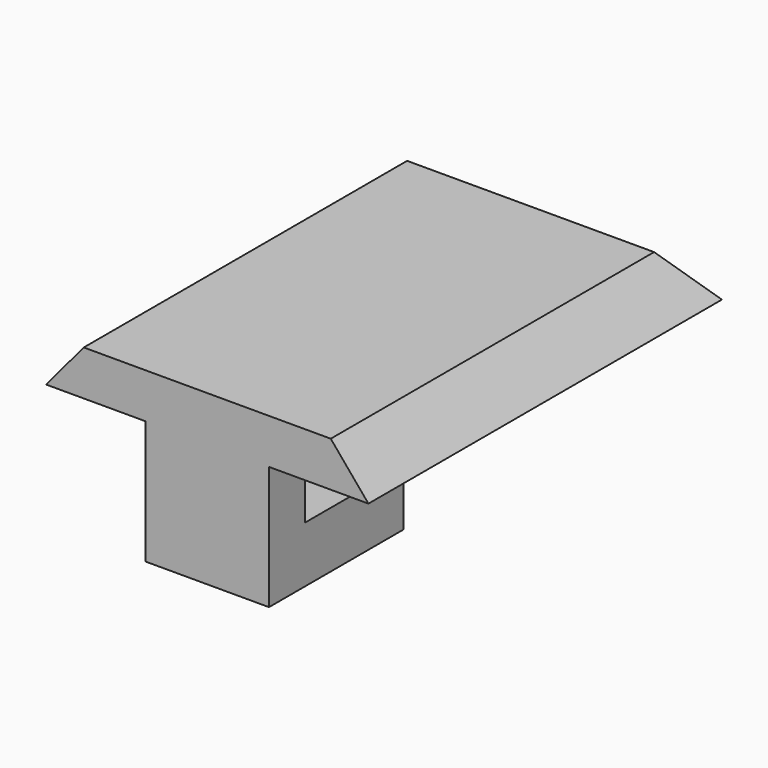
from build123d import *

# Parameters (mm, degrees)
F1_DEPTH    = 5.5
F2_DEPTH    = 15
F3_T1_DEPTH = 64.5730638659
F3_T3_DEPTH = 54.5730638659


# Not quite as in the source:
# - a fillet or chamfer that OpenCascade refuses, or shapes differently, is made with other operations: its cross-section is extruded or revolved along the edge and cut away or added


with BuildPart() as f1:
    # F0 (on Right) → F1 (new body, symmetric)
    with BuildSketch(Plane.YZ):
        Polygon((-11, 0), (0, 0), (0, 5), (-11, 5), (-11, 11), (-15, 11), (-15, 0), align=None)
    extrude(amount=F1_DEPTH, both=True)

    # F0 (on Right) → F2 (join, symmetric)
    with BuildSketch(Plane.YZ):
        Polygon((-15, 15), (-15, 11), (-11, 11), (25, 11), (25, 15), align=None)
    extrude(amount=F2_DEPTH, both=True)

    # F3: chamfer of 4 x 4.7670143704 on 3 edges, made by hand

    # F3_s2 → F3_t1 (cut)
    with BuildSketch(Plane.XZ.offset(-37.2865319329)):
        Polygon((15, 10.2329856296), (11, 15), (15, 15), align=None)
        Polygon((-15, 10.2329856296), (-11, 15), (-15, 15), align=None)
    extrude(amount=F3_T1_DEPTH, mode=Mode.SUBTRACT)

    # F3_s4 → F3_t3 (cut)
    with BuildSketch(Plane.YZ.offset(-27.2865319329)):
        Polygon((21, 15), (25, 10.2329856296), (25, 15), align=None)
    extrude(amount=F3_T3_DEPTH, mode=Mode.SUBTRACT)


solid = f1.part
